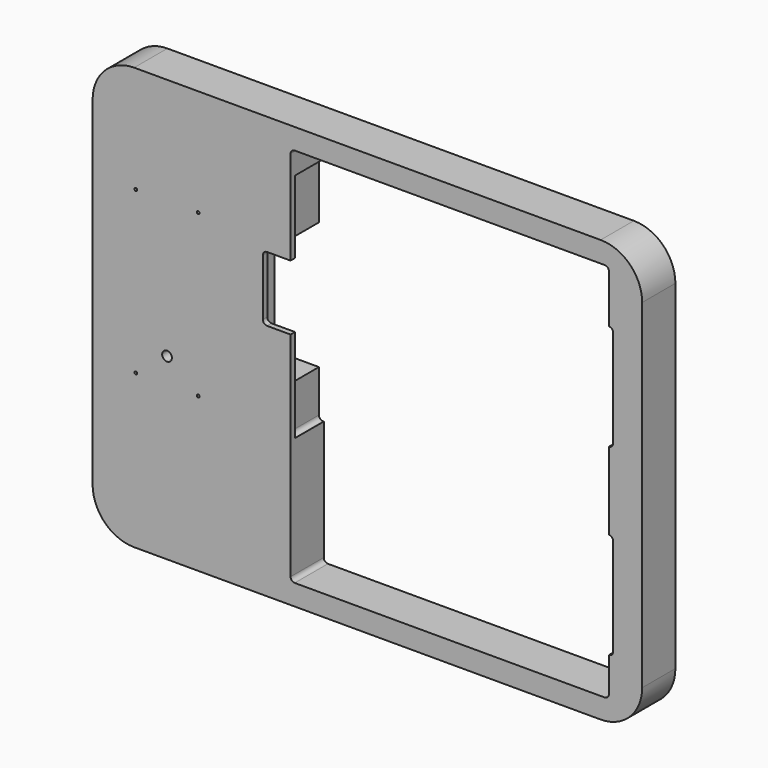
from build123d import *

# Parameters (mm, degrees)
F0_W      = 397
F0_H      = 305
F1_DEPTH  = 30
F2_W      = 230
F2_H      = 275
F3_DEPTH  = 30
F4_R      = 3
F5_R      = 30
F6_W      = 26
F6_H      = 167
F7_DEPTH  = 3.5
F8_R      = 3
F10_W     = 32
F10_H     = 92
F11_DEPTH = 26
F12_R     = 3
F13_W     = 4
F13_H     = 47
F14_DEPTH = 20
F15_R     = 3
F16_W     = 30
F16_H     = 76.5
F17_DEPTH = 3
F18_R     = 2.99999
F19_R     = 3.5
F20_DEPTH = 30
F21_W     = 99
F21_H     = 62
F22_DEPTH = 18
F23_R     = 3
F25_DEPTH = 6
F26_W     = 13
F26_H     = 20
F26_H_2   = 6
F27_DEPTH = 30
F28_R     = 1
F29_DEPTH = 30
F31_DEPTH = 20


# Not quite as in the source:
# - a fillet or chamfer is up to 0.001 mm smaller than in the source, because OpenCascade refuses the exact size
# - a feature names something its author has since deleted; it is built from what else it names


with BuildPart() as f1:
    # F0 (on Front) → F1 (new body)
    with BuildSketch(Plane.XZ):
        with Locations((0, 5)):
            Rectangle(F0_W, F0_H)
    extrude(amount=F1_DEPTH)

    # F2 (on face) → F3 (cut, through all)
    with BuildSketch(Plane.XZ.offset(30)):
        with Locations((59.5, 5)):
            Rectangle(F2_W, F2_H)
    extrude(amount=-F3_DEPTH, mode=Mode.SUBTRACT)

    # F4
    f4_edges = [f1.edges().sort_by_distance(p)[0] for p in [
        (-55.5, -15, 142.5),
        (174.5, -15, 142.5),
        (174.5, -15, -132.5),
        (-55.5, -15, -132.5),
    ]]
    fillet(f4_edges, radius=F4_R)

    # F5
    f5_edges = [f1.edges().sort_by_distance(p)[0] for p in [
        (-198.5, -15, -147.5),
        (-198.5, -15, 157.5),
        (198.5, -15, 157.5),
        (198.5, -15, -147.5),
    ]]
    fillet(f5_edges, radius=F5_R)

    # F6 (on face) → F7 (cut)
    with BuildSketch(Plane.YZ.offset(-55.5)):
        with Locations((-13, 40.5)):
            Rectangle(F6_W, F6_H)
    extrude(amount=-F7_DEPTH, mode=Mode.SUBTRACT)

    # F8
    f8_edges = [f1.edges().sort_by_distance(p)[0] for p in [
        (-59, -13, -43),
        (-59, -13, 124),
    ]]
    fillet(f8_edges, radius=F8_R)

    # F10 (on face) → F11 (cut)
    with BuildSketch(Plane(origin=(0, 0, 0), x_dir=(-1, 0, 0), z_dir=(0, 1, 0))):
        with Locations((75, 36.5)):
            Rectangle(F10_W, F10_H)
    extrude(amount=-F11_DEPTH, mode=Mode.SUBTRACT)

    # F12
    f12_edges = [f1.edges().sort_by_distance(p)[0] for p in [
        (-91, -13, -9.5),
        (-91, -13, 82.5),
    ]]
    fillet(f12_edges, radius=F12_R)

    # F13 (on face) → F14 (cut)
    with BuildSketch(Plane.YZ.offset(-55.5)):
        with Locations((-28, 48)):
            Rectangle(F13_W, F13_H)
    extrude(amount=-F14_DEPTH, mode=Mode.SUBTRACT)

    # F15
    f15_edges = [f1.edges().sort_by_distance(p)[0] for p in [
        (-75.5, -28, 24.5),
        (-75.5, -28, 71.5),
    ]]
    fillet(f15_edges, radius=F15_R)

    # F16 (on face) → F17 (cut)
    with BuildSketch(Plane(origin=(174.5, 0, 0), x_dir=(0, -1, 0), z_dir=(-1, 0, 0))):
        with Locations((15, -66.25)):
            Rectangle(F16_W, F16_H)
        with Locations((15, 66.25)):
            Rectangle(F16_W, F16_H)
    extrude(amount=-F17_DEPTH, mode=Mode.SUBTRACT)

    # F18 (radius 3 in the source; OpenCascade refuses exactly that, so slightly less here)
    f18_edges = [f1.edges().sort_by_distance(p)[0] for p in [
        (177.5, -15, -104.5),
        (177.5, -15, 28),
        (177.5, -15, 104.5),
        (177.5, -15, -28),
    ]]
    fillet(f18_edges, radius=F18_R)

    # F19 (on face) → F20 (cut)
    with BuildSketch(Plane.XZ.offset(30)):
        with Locations((-144.75, -18.25)):
            Circle(F19_R)
    extrude(amount=-F20_DEPTH, mode=Mode.SUBTRACT)

    # F21 (on face) → F22 (cut)
    with BuildSketch(Plane(origin=(0, 0, 0), x_dir=(-1, 0, 0), z_dir=(0, 1, 0))):
        with Locations((119, -92.75)):
            Rectangle(F21_W, F21_H)
    extrude(amount=-F22_DEPTH, mode=Mode.SUBTRACT)

    # F23
    f23_edges = [f1.edges().sort_by_distance(p)[0] for p in [
        (-168.5, -9, -123.75),
        (-69.5, -9, -123.75),
        (-69.5, -9, -61.75),
        (-168.5, -9, -61.75),
    ]]
    fillet(f23_edges, radius=F23_R)

    # F24 (on face) → F25 (cut)
    with BuildSketch(Plane(origin=(0, 0, 0), x_dir=(-1, 0, 0), z_dir=(0, 1, 0))):
        with BuildLine():
            ThreePointArc((148.25, -18.25), (144.75, -21.75), (141.25, -18.25))
            Line((141.25, -18.25), (141.25, -61.75))
            Line((141.25, -61.75), (148.25, -61.75))
            Line((148.25, -61.75), (148.25, -18.25))
        make_face()
    extrude(amount=-F25_DEPTH, mode=Mode.SUBTRACT)

    # F26 (on face) → F27 (cut)
    with BuildSketch(Plane(origin=(-198.5, 0, 0), x_dir=(0, -1, 0), z_dir=(-1, 0, 0))):
        with Locations((6.5, -87.5)):
            Rectangle(F26_W, F26_H)
        with Locations((6.5, -108.5)):
            Rectangle(F26_W, F26_H_2)
    extrude(amount=-F27_DEPTH, mode=Mode.SUBTRACT)

    # F28 (on face) → F29 (cut)
    with BuildSketch(Plane.XZ.offset(30)):
        with Locations((-167.25, 80.35)):
            Circle(F28_R)
        with Locations((-167.25, -36.25)):
            Circle(F28_R)
        with Locations((-122.25, -36.25)):
            Circle(F28_R)
        with Locations((-122.25, 80.35)):
            Circle(F28_R)
    extrude(amount=-F29_DEPTH, mode=Mode.SUBTRACT)

    # F30 (on face) → F31 (cut)
    with BuildSketch(Plane(origin=(0, 0, 0), x_dir=(-1, 0, 0), z_dir=(0, 1, 0))):
        with BuildLine():
            Line((-186.5, 125), (-186.5, 127))
            ThreePointArc((-186.5, 127), (-187.5, 126), (-186.5, 125))
        make_face()
        with BuildLine():
            ThreePointArc((-185.5, 126), (-185.7928932188, 126.7071067812), (-186.5, 127))
            Line((-186.5, 127), (-186.5, 125))
            ThreePointArc((-186.5, 125), (-185.7928932188, 125.2928932188), (-185.5, 126))
        make_face()
        with BuildLine():
            ThreePointArc((-60.5, 150), (-59.5, 149), (-58.5, 150))
            Line((-58.5, 150), (-60.5, 150))
        make_face()
        with BuildLine():
            Line((-60.5, 150), (-58.5, 150))
            ThreePointArc((-58.5, 150), (-59.5, 151), (-60.5, 150))
        make_face()
        with BuildLine():
            Line((140.25, 150), (142.25, 150))
            ThreePointArc((142.25, 150), (141.25, 151), (140.25, 150))
        make_face()
        with BuildLine():
            ThreePointArc((140.25, 150), (141.25, 149), (142.25, 150))
            Line((142.25, 150), (140.25, 150))
        make_face()
        with BuildLine():
            ThreePointArc((187.5, 5), (187.2071067812, 5.7071067812), (186.5, 6))
            Line((186.5, 6), (186.5, 4))
            ThreePointArc((186.5, 4), (187.2071067812, 4.2928932188), (187.5, 5))
        make_face()
        with BuildLine():
            Line((186.5, 4), (186.5, 6))
            ThreePointArc((186.5, 6), (185.5, 5), (186.5, 4))
        make_face()
        with BuildLine():
            Line((140.25, -140), (142.25, -140))
            ThreePointArc((142.25, -140), (141.25, -139), (140.25, -140))
        make_face()
        with BuildLine():
            ThreePointArc((140.25, -140), (141.25, -141), (142.25, -140))
            Line((142.25, -140), (140.25, -140))
        make_face()
        with BuildLine():
            Line((-60.5, -140), (-58.5, -140))
            ThreePointArc((-58.5, -140), (-59.5, -139), (-60.5, -140))
        make_face()
        with BuildLine():
            ThreePointArc((-60.5, -140), (-59.5, -141), (-58.5, -140))
            Line((-58.5, -140), (-60.5, -140))
        make_face()
        with BuildLine():
            ThreePointArc((-185.5, -116), (-185.7928932188, -115.2928932188), (-186.5, -115))
            Line((-186.5, -115), (-186.5, -117))
            ThreePointArc((-186.5, -117), (-185.7928932188, -116.7071067812), (-185.5, -116))
        make_face()
        with BuildLine():
            Line((-186.5, -117), (-186.5, -115))
            ThreePointArc((-186.5, -115), (-187.5, -116), (-186.5, -117))
        make_face()
        with BuildLine():
            Line((-186.5, 4), (-186.5, 6))
            ThreePointArc((-186.5, 6), (-187.5, 5), (-186.5, 4))
        make_face()
        with BuildLine():
            ThreePointArc((-185.5, 5), (-185.7928932188, 5.7071067812), (-186.5, 6))
            Line((-186.5, 6), (-186.5, 4))
            ThreePointArc((-186.5, 4), (-185.7928932188, 4.2928932188), (-185.5, 5))
        make_face()
    extrude(amount=-F31_DEPTH, mode=Mode.SUBTRACT)


solid = f1.part
